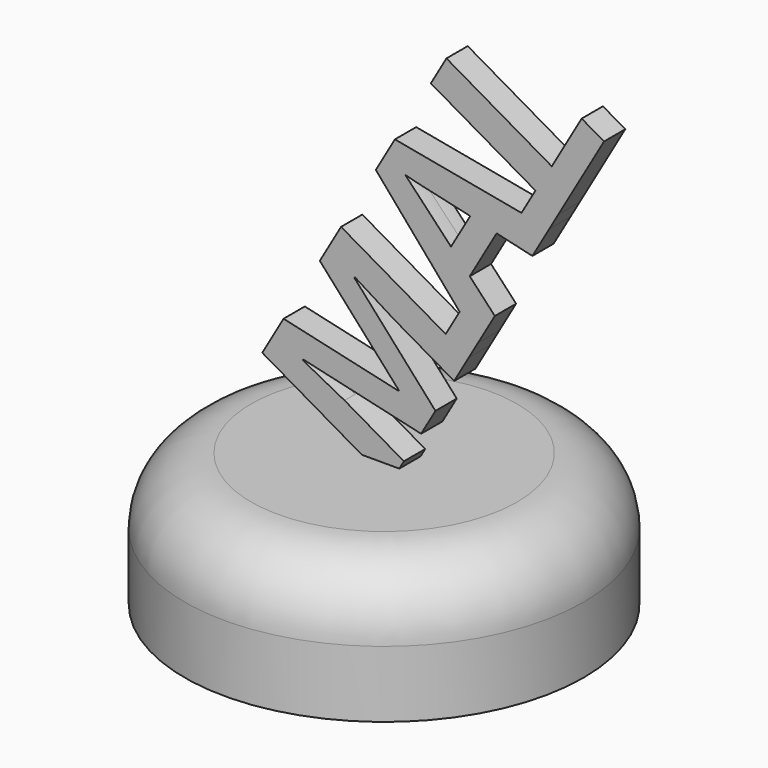
from build123d import *

# Parameters (mm, degrees)
F0_R           = 30
F1_DEPTH       = 20
F2_R           = 10
F3_TEXT_SIZE   = 31.0519658443
F4_DEPTH       = 2
F5_W           = 4
F5_H           = 5.1793053594
F5_H_2         = 3.9566822502
F6_DEPTH       = 4
F7_W           = 4
F7_H           = 7.3733483229
F8_DEPTH       = 4
F9_TEXT_SIZE   = 3.255744837
F9_TEXT_SIZE_2 = 4.6615519083
F10_DEPTH      = 3


# Not quite as in the source:
# - Text() gives the source's letters only with a copy of the font that has no kerning and outlines rounded to 1/6400 em; it was checked with that copy


with BuildPart() as f1:
    # F0 (on Top) → F1 (new body)
    with BuildSketch(Plane.XY):
        Circle(F0_R)
    extrude(amount=F1_DEPTH)

    # F2
    f2_edges = [f1.edges().sort_by_distance(p)[0] for p in [
        (-30, 0, 20),
    ]]
    fillet(f2_edges, radius=F2_R)

    # F3 (on Front) → F4 (join, symmetric)
    with BuildSketch(Plane.XZ):
        with Locations(Location((1.0754619725, 15.1427984238), (0, 0, 60))):
            Text('MAL', F3_TEXT_SIZE, font='Open Sans', font_style=FontStyle.BOLD, text_align=(TextAlign.LEFT, TextAlign.BOTTOM))
    extrude(amount=F4_DEPTH, both=True)

    # F5 (on face) → F6 (join)
    with BuildSketch(Plane(origin=(-5.7504275803, 0, 3.3200109114), x_dir=(0, 1, 0), z_dir=(0.8660254038, 0, -0.5))):
        with Locations((0, 64.5539894624)):
            Rectangle(F5_W, F5_H)
        with Locations((0, 69.1219832672)):
            Rectangle(F5_W, F5_H_2)
    extrude(amount=-F6_DEPTH)

    # F7 (on face) → F8 (join)
    with BuildSketch(Plane(origin=(-5.7504275803, 0, 3.3200109114), x_dir=(0, 1, 0), z_dir=(0.8660254038, 0, -0.5))):
        with Locations((0, 41.6341906054)):
            Rectangle(F7_W, F7_H)
    extrude(amount=-F8_DEPTH)

    # F9 (on face) → F10 (cut)
    with BuildSketch(Plane(origin=(0, 0, 0), x_dir=(1, 0, 0), z_dir=(0, 0, -1))):
        with Locations((-6.5159267905, 0)):
            Text('you lost', F9_TEXT_SIZE, font='Open Sans', font_style=FontStyle.BOLD, text_align=(TextAlign.LEFT, TextAlign.BOTTOM))
        with Locations((-15.0837351732, -5.3643704394)):
            Text('Luke is great', F9_TEXT_SIZE_2, font='Open Sans', font_style=FontStyle.BOLD, text_align=(TextAlign.LEFT, TextAlign.BOTTOM))
    extrude(amount=-F10_DEPTH, mode=Mode.SUBTRACT)


solid = f1.part
